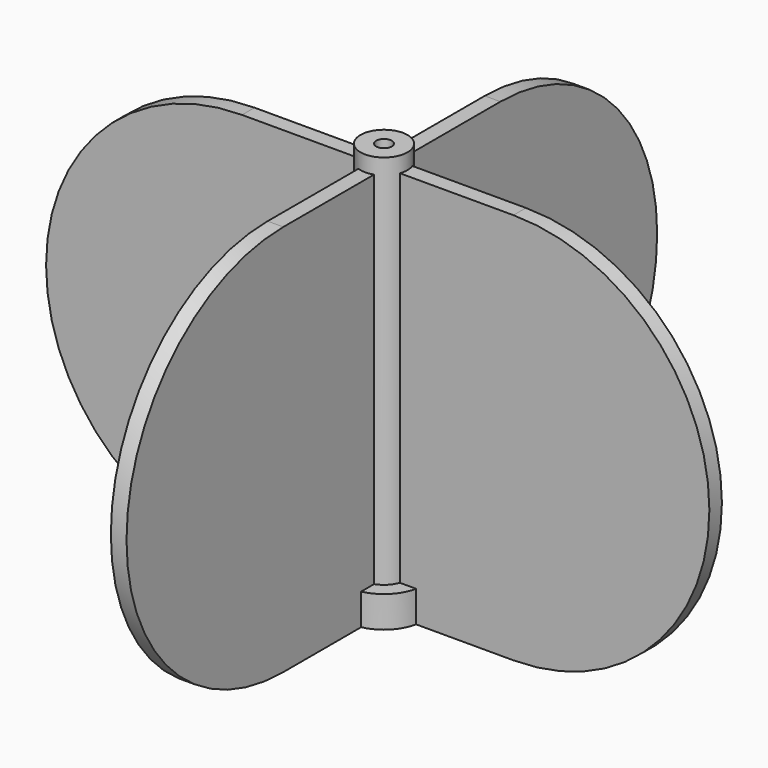
from build123d import *
from build123d import SkipClean  # not in build123d's __all__

# Parameters (mm, degrees)
F1_DEPTH  = 25
F2_R      = 0.5
F3_DEPTH  = 1
F4_R      = 2.5
F4_R_2    = 0.5
F5_DEPTH  = 2
F7_DEPTH  = 1
F9_DEPTH  = 1
F11_DEPTH = 1
F12_DEPTH = 1
F14_DEPTH = 1


# Not quite as in the source:
# - a feature names something its author has since deleted; it is built from what else it names


with BuildPart() as f1:
    # F0 (on Top) → F1 (new body)
    with BuildSketch(Plane.XY):
        with BuildLine():
            Line((-8.65676943, -0.5), (-1.4142135624, -0.5))
            ThreePointArc((-1.4142135624, -0.5), (-1.0606601718, -1.0606601718), (-0.5, -1.4142135624))
            Line((-0.5, -1.4142135624), (-0.5, -8.65676943))
            Line((-0.5, -8.65676943), (0.5, -8.65676943))
            Line((0.5, -8.65676943), (0.5, -1.4142135624))
            ThreePointArc((0.5, -1.4142135624), (1.0606601718, -1.0606601718), (1.4142135624, -0.5))
            Line((1.4142135624, -0.5), (8.65676943, -0.5))
            Line((8.65676943, -0.5), (8.65676943, 0.5))
            Line((8.65676943, 0.5), (1.4142135624, 0.5))
            ThreePointArc((1.4142135624, 0.5), (1.0606601718, 1.0606601718), (0.5, 1.4142135624))
            Line((0.5, 1.4142135624), (0.5, 8.65676943))
            Line((0.5, 8.65676943), (-0.5, 8.65676943))
            Line((-0.5, 8.65676943), (-0.5, 1.4142135624))
            ThreePointArc((-0.5, 1.4142135624), (-1.0606601718, 1.0606601718), (-1.4142135624, 0.5))
            Line((-1.4142135624, 0.5), (-8.65676943, 0.5))
            Line((-8.65676943, 0.5), (-8.65676943, -0.5))
        make_face()
        with BuildLine():
            ThreePointArc((0, 0.5), (0.3535533906, 0.3535533906), (0.5, 0))
            ThreePointArc((0.5, 0), (-0.3535533906, -0.3535533906), (0, 0.5))
        make_face(mode=Mode.SUBTRACT)
    extrude(amount=F1_DEPTH)

    # F2 (on face) → F3 (join)
    with BuildSketch(Plane.XY.offset(25)):
        with BuildLine():
            ThreePointArc((1.4142135624, -0.5), (1.4783978395, -0.2536529681), (1.5, 0))
            ThreePointArc((1.5, 0), (1.4783978395, 0.2536529681), (1.4142135624, 0.5))
            ThreePointArc((1.4142135624, 0.5), (1.0606601718, 1.0606601718), (0.5, 1.4142135624))
            ThreePointArc((0.5, 1.4142135624), (0, 1.5), (-0.5, 1.4142135624))
            ThreePointArc((-0.5, 1.4142135624), (-1.0606601718, 1.0606601718), (-1.4142135624, 0.5))
            ThreePointArc((-1.4142135624, 0.5), (-1.5, 0), (-1.4142135624, -0.5))
            ThreePointArc((-1.4142135624, -0.5), (-1.0606601718, -1.0606601718), (-0.5, -1.4142135624))
            ThreePointArc((-0.5, -1.4142135624), (0, -1.5), (0.5, -1.4142135624))
            ThreePointArc((0.5, -1.4142135624), (1.0606601718, -1.0606601718), (1.4142135624, -0.5))
        make_face()
        Circle(F2_R, mode=Mode.SUBTRACT)
    with SkipClean():  # cleaning this boolean's faces spoils the solid; the shape is the same uncleaned
        extrude(amount=F3_DEPTH)

    # F4 (on face) → F5 (join)
    with BuildSketch(Plane(origin=(0, 0, 0), x_dir=(1, 0, 0), z_dir=(0, 0, -1))):
        Circle(F4_R)
        Circle(F4_R_2, mode=Mode.SUBTRACT)
    extrude(amount=-F5_DEPTH)

    # F6 (on face) → F7 (join)
    with BuildSketch(Plane.YZ.offset(0.5)):
        with BuildLine():
            Line((-8.65676943, 0), (-8.65676943, 25))
            ThreePointArc((-8.65676943, 25), (-21.15676943, 12.5), (-8.65676943, 0))
        make_face()
    extrude(amount=-F7_DEPTH)

    # F8 (on face) → F9 (join)
    with BuildSketch(Plane(origin=(0, 0.5, 0), x_dir=(-1, 0, 0), z_dir=(0, 1, 0))):
        with BuildLine():
            Line((8.65676943, 25), (8.65676943, 0))
            ThreePointArc((8.65676943, 0), (21.15676943, 12.5), (8.65676943, 25))
        make_face()
    extrude(amount=-F9_DEPTH)

    # F10 (on face) → F11 (join)
    with BuildSketch(Plane(origin=(-0.5, 0, 0), x_dir=(0, -1, 0), z_dir=(-1, 0, 0))):
        with BuildLine():
            Line((-8.65676943, 0), (-8.65676943, 25))
            ThreePointArc((-8.65676943, 25), (-21.15676943, 12.5), (-8.65676943, 0))
        make_face()
    extrude(amount=-F11_DEPTH)


with BuildPart() as f12:
    # F12 (new): a face of the model
    f12_faces = [f1.part.faces().sort_by_distance(p)[0] for p in [
        (5.0713936624, 0.5, 12.63302926),
    ]]
    extrude(f12_faces, amount=-F12_DEPTH)


with BuildPart() as f1_1:
    add(f1.part, clean=False)

    add(f12.part)  # F14 merges F12
    # F13 (on face) → F14 (join)
    with BuildSketch(Plane(origin=(0, 0.5, 0), x_dir=(-1, 0, 0), z_dir=(0, 1, 0))):
        with BuildLine():
            Line((-8.65676943, 0), (-8.65676943, 25))
            ThreePointArc((-8.65676943, 25), (-21.15676943, 12.5), (-8.65676943, 0))
        make_face()
    extrude(amount=-F14_DEPTH)


solid = f1_1.part
